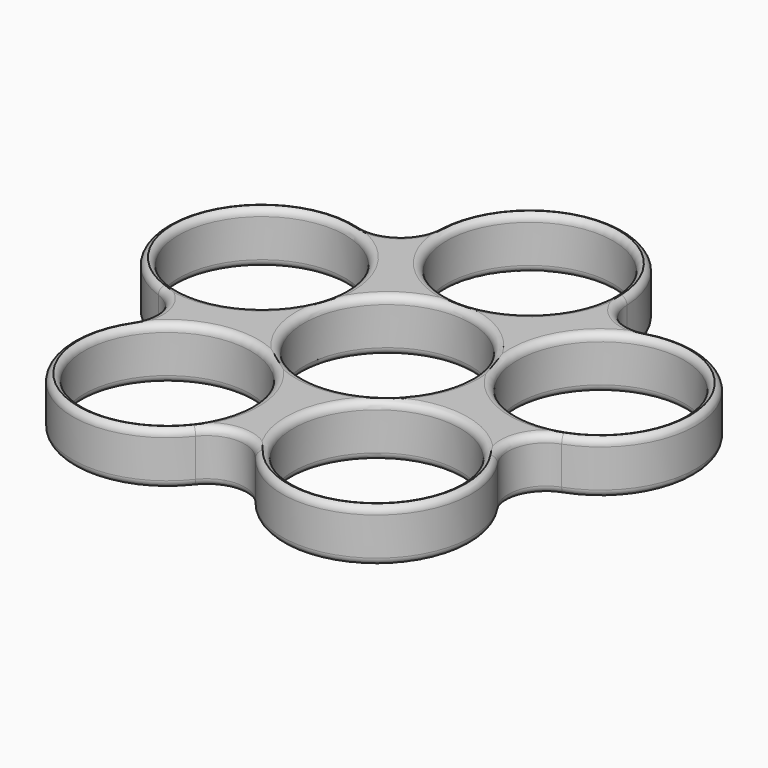
from build123d import *

# Parameters (mm, degrees)
F0_R         = 11
F1_DEPTH     = 7
F2_T3_ANGLE  = 176.2424563909
F2_T6_ANGLE  = 176.2424563909
F2_T45_ANGLE = 104.2424563909
F2_T48_ANGLE = 104.2424563909
F2_T51_ANGLE = 176.2424563909
F2_T54_ANGLE = 104.2424563909
F2_T57_ANGLE = 176.2424563909
F2_T60_ANGLE = 104.2424563909
F2_T63_ANGLE = 176.2424563909
F2_T66_ANGLE = 104.2424563909
F2_T69_ANGLE = 176.2424563909
F2_T72_ANGLE = 104.2424563909
F2_T75_ANGLE = 104.2424563909
F2_T78_ANGLE = 176.2424563909
F2_T81_ANGLE = 104.2424563909
F2_T84_ANGLE = 176.2424563909
F2_T87_ANGLE = 104.2424563909
F2_T90_ANGLE = 176.2424563909
F2_T93_ANGLE = 104.2424563909
F2_T96_ANGLE = 176.2424563909


# Not quite as in the source:
# - a fillet or chamfer that OpenCascade refuses, or shapes differently, is made with other operations: its cross-section is extruded or revolved along the edge and cut away or added


with BuildPart() as f1:
    # F0 (on Top) → F1 (new body)
    with BuildSketch(Plane.XY):
        with BuildLine():
            ThreePointArc((18.8789455733, 19.2703536504), (14.551666288, 20.0286503916), (12.4932803925, 23.9098109739))
            ThreePointArc((12.4932803925, 23.9098109739), (0, 36), (-12.4932803925, 23.9098109739))
            ThreePointArc((-12.4932803925, 23.9098109739), (-14.551666288, 20.0286503916), (-18.8789455733, 19.2703536504))
            ThreePointArc((-18.8789455733, 19.2703536504), (-34.2380345866, 11.1246117975), (-26.6002174869, -4.493277804))
            ThreePointArc((-26.6002174869, -4.493277804), (-23.545090647, -7.6502637008), (-24.1611104286, -12.0000774427))
            ThreePointArc((-24.1611104286, -12.0000774427), (-21.1602690825, -29.1246117975), (-3.9465581225, -26.6868093776))
            ThreePointArc((-3.9465581225, -26.6868093776), (0, -24.7567733816), (3.9465581225, -26.6868093776))
            ThreePointArc((3.9465581225, -26.6868093776), (21.1602690825, -29.1246117975), (24.1611104286, -12.0000774427))
            ThreePointArc((24.1611104286, -12.0000774427), (23.545090647, -7.6502637008), (26.6002174869, -4.493277804))
            ThreePointArc((26.6002174869, -4.493277804), (34.2380345866, 11.1246117975), (18.8789455733, 19.2703536504))
        make_face()
        with Locations((-13.8129534289, -19.0118993678)):
            Circle(F0_R, mode=Mode.SUBTRACT)
        with Locations((13.8129534289, -19.0118993678)):
            Circle(F0_R, mode=Mode.SUBTRACT)
        Circle(F0_R, mode=Mode.SUBTRACT)
        with Locations((-22.3498281329, 7.2618993678)):
            Circle(F0_R, mode=Mode.SUBTRACT)
        with Locations((22.3498281329, 7.2618993678)):
            Circle(F0_R, mode=Mode.SUBTRACT)
        with Locations((0, 23.5)):
            Circle(F0_R, mode=Mode.SUBTRACT)
    extrude(amount=F1_DEPTH)

    # F2: fillet of radius 1 on 14 edges, made by hand


with BuildPart() as f2_tool1:
    # F2_s2 → F2_t3 (revolve)
    with BuildSketch(Plane(origin=(-22.5637579595, 6.5217514376, 0), x_dir=(0, 0, 1), z_dir=(0.9606763426, -0.2776706048, 0))):
        with BuildLine():
            ThreePointArc((6, -13.2704446309), (6.7071067812, -12.9775514121), (7, -12.2704446309))
            Line((7, -12.2704446309), (7, -13.2704446309))
            Line((7, -13.2704446309), (6, -13.2704446309))
        make_face()
    revolve(axis=Axis((-22.3498281329, 7.2618993678, 7), (0, 0, 1)), revolution_arc=F2_T3_ANGLE)


with BuildPart() as f2_tool4:
    # F2_s5 → F2_t6 (revolve)
    with BuildSketch(Plane(origin=(-13.1751388688, -19.4440770122, 0), x_dir=(0, 0, 1), z_dir=(0.560945754, 0.82785256, 0))):
        with BuildLine():
            ThreePointArc((1, -13.2704446309), (0.2928932188, -12.9775514121), (0, -12.2704446309))
            Line((0, -12.2704446309), (0, -13.2704446309))
            Line((0, -13.2704446309), (1, -13.2704446309))
        make_face()
    revolve(axis=Axis((-13.8129534289, -19.0118993678, 0), (0, 0, 1)), revolution_arc=F2_T6_ANGLE)


with BuildPart() as f2_tool7:
    # F2_s8 → F2_t9 (revolve)
    with BuildSketch(Plane.XZ.offset(19.0118993678)):
        with BuildLine():
            ThreePointArc((-2.8129534289, 6), (-2.5200602101, 6.7071067812), (-1.8129534289, 7))
            Line((-1.8129534289, 7), (-2.8129534289, 7))
            Line((-2.8129534289, 7), (-2.8129534289, 6))
        make_face()
    revolve(axis=Axis((-13.8129534289, -19.0118993678, 7), (0, 0, 1)))


with BuildPart() as f2_tool10:
    # F2_s11 → F2_t12 (revolve)
    with BuildSketch(Plane.XZ.offset(-7.2618993678)):
        with BuildLine():
            ThreePointArc((-11.3498281329, 6), (-11.0569349141, 6.7071067812), (-10.3498281329, 7))
            Line((-10.3498281329, 7), (-11.3498281329, 7))
            Line((-11.3498281329, 7), (-11.3498281329, 6))
        make_face()
    revolve(axis=Axis((-22.3498281329, 7.2618993678, 7), (0, 0, 1)))


with BuildPart() as f2_tool13:
    # F2_s14 → F2_t15 (revolve)
    with BuildSketch(Plane.XZ.offset(-23.5)):
        with BuildLine():
            ThreePointArc((11, 1), (11.2928932188, 0.2928932188), (12, 0))
            Line((12, 0), (11, 0))
            Line((11, 0), (11, 1))
        make_face()
    revolve(axis=Axis((0, 23.5, 0), (0, 0, 1)))


with BuildPart() as f2_tool16:
    # F2_s17 → F2_t18 (revolve)
    with BuildSketch(Plane.XZ.offset(-23.5)):
        with BuildLine():
            ThreePointArc((11, 6), (11.2928932188, 6.7071067812), (12, 7))
            Line((12, 7), (11, 7))
            Line((11, 7), (11, 6))
        make_face()
    revolve(axis=Axis((0, 23.5, 7), (0, 0, 1)))


with BuildPart() as f2_tool19:
    # F2_s20 → F2_t21 (revolve)
    with BuildSketch(Plane.XZ.offset(-7.2618993678)):
        with BuildLine():
            ThreePointArc((-11.3498281329, 1), (-11.0569349141, 0.2928932188), (-10.3498281329, 0))
            Line((-10.3498281329, 0), (-11.3498281329, 0))
            Line((-11.3498281329, 0), (-11.3498281329, 1))
        make_face()
    revolve(axis=Axis((-22.3498281329, 7.2618993678, 0), (0, 0, 1)))


with BuildPart() as f2_tool22:
    # F2_s23 → F2_t24 (revolve)
    with BuildSketch(Plane.XZ.offset(19.0118993678)):
        with BuildLine():
            ThreePointArc((-2.8129534289, 1), (-2.5200602101, 0.2928932188), (-1.8129534289, 0))
            Line((-1.8129534289, 0), (-2.8129534289, 0))
            Line((-2.8129534289, 0), (-2.8129534289, 1))
        make_face()
    revolve(axis=Axis((-13.8129534289, -19.0118993678, 0), (0, 0, 1)))


with BuildPart() as f2_tool25:
    # F2_s26 → F2_t27 (revolve)
    with BuildSketch(Plane.XZ):
        with BuildLine():
            ThreePointArc((11, 1), (11.2928932188, 0.2928932188), (12, 0))
            Line((12, 0), (11, 0))
            Line((11, 0), (11, 1))
        make_face()
    revolve(axis=Axis((0, 0, 0), (0, 0, 1)))


with BuildPart() as f2_tool28:
    # F2_s29 → F2_t30 (revolve)
    with BuildSketch(Plane.XZ):
        with BuildLine():
            ThreePointArc((11, 6), (11.2928932188, 6.7071067812), (12, 7))
            Line((12, 7), (11, 7))
            Line((11, 7), (11, 6))
        make_face()
    revolve(axis=Axis((0, 0, 7), (0, 0, 1)))


with BuildPart() as f2_tool31:
    # F2_s32 → F2_t33 (revolve)
    with BuildSketch(Plane.XZ.offset(-7.2618993678)):
        with BuildLine():
            ThreePointArc((33.3498281329, 1), (33.6427213517, 0.2928932188), (34.3498281329, 0))
            Line((34.3498281329, 0), (33.3498281329, 0))
            Line((33.3498281329, 0), (33.3498281329, 1))
        make_face()
    revolve(axis=Axis((22.3498281329, 7.2618993678, 0), (0, 0, 1)))


with BuildPart() as f2_tool34:
    # F2_s35 → F2_t36 (revolve)
    with BuildSketch(Plane.XZ.offset(-7.2618993678)):
        with BuildLine():
            ThreePointArc((33.3498281329, 6), (33.6427213517, 6.7071067812), (34.3498281329, 7))
            Line((34.3498281329, 7), (33.3498281329, 7))
            Line((33.3498281329, 7), (33.3498281329, 6))
        make_face()
    revolve(axis=Axis((22.3498281329, 7.2618993678, 7), (0, 0, 1)))


with BuildPart() as f2_tool37:
    # F2_s38 → F2_t39 (revolve)
    with BuildSketch(Plane.XZ.offset(19.0118993678)):
        with BuildLine():
            ThreePointArc((24.8129534289, 1), (25.1058466477, 0.2928932188), (25.8129534289, 0))
            Line((25.8129534289, 0), (24.8129534289, 0))
            Line((24.8129534289, 0), (24.8129534289, 1))
        make_face()
    revolve(axis=Axis((13.8129534289, -19.0118993678, 0), (0, 0, 1)))


with BuildPart() as f2_tool40:
    # F2_s41 → F2_t42 (revolve)
    with BuildSketch(Plane.XZ.offset(19.0118993678)):
        with BuildLine():
            ThreePointArc((24.8129534289, 6), (25.1058466477, 6.7071067812), (25.8129534289, 7))
            Line((25.8129534289, 7), (24.8129534289, 7))
            Line((24.8129534289, 7), (24.8129534289, 6))
        make_face()
    revolve(axis=Axis((13.8129534289, -19.0118993678, 7), (0, 0, 1)))


with BuildPart() as f2_tool43:
    # F2_s44 → F2_t45 (revolve)
    with BuildSketch(Plane(origin=(-22.0878529604, 7.9864364188, 0), x_dir=(0, 0, 1), z_dir=(-0.9404141737, 0.3400311483, 0))):
        with BuildLine():
            ThreePointArc((1, -13.2704446309), (0.2928932188, -12.9775514121), (0, -12.2704446309))
            Line((0, -12.2704446309), (0, -13.2704446309))
            Line((0, -13.2704446309), (1, -13.2704446309))
        make_face()
    revolve(axis=Axis((-28.3003732285, -9.1953486727, 0), (0, 0, -1)), revolution_arc=F2_T45_ANGLE)


with BuildPart() as f2_tool46:
    # F2_s47 → F2_t48 (revolve)
    with BuildSketch(Plane(origin=(-14.4210743321, -18.538851911, 0), x_dir=(0, 0, 1), z_dir=(-0.6139928008, -0.7893116245, 0))):
        with BuildLine():
            ThreePointArc((1, -13.2704446309), (0.2928932188, -12.9775514121), (0, -12.2704446309))
            Line((0, -12.2704446309), (0, -13.2704446309))
            Line((0, -13.2704446309), (1, -13.2704446309))
        make_face()
    revolve(axis=Axis((0, -29.7567733816, 0), (0, 0, -1)), revolution_arc=F2_T48_ANGLE)


with BuildPart() as f2_tool49:
    # F2_s50 → F2_t51 (revolve)
    with BuildSketch(Plane(origin=(14.4210743321, -18.538851911, 0), x_dir=(0, 0, 1), z_dir=(-0.6139928008, 0.7893116245, 0))):
        with BuildLine():
            ThreePointArc((1, -13.2704446309), (0.2928932188, -12.9775514121), (0, -12.2704446309))
            Line((0, -12.2704446309), (0, -13.2704446309))
            Line((0, -13.2704446309), (1, -13.2704446309))
        make_face()
    revolve(axis=Axis((13.8129534289, -19.0118993678, 0), (0, 0, 1)), revolution_arc=F2_T51_ANGLE)


with BuildPart() as f2_tool52:
    # F2_s53 → F2_t54 (revolve)
    with BuildSketch(Plane(origin=(13.1751388688, -19.4440770122, 0), x_dir=(0, 0, 1), z_dir=(0.560945754, -0.82785256, 0))):
        with BuildLine():
            ThreePointArc((1, -13.2704446309), (0.2928932188, -12.9775514121), (0, -12.2704446309))
            Line((0, -12.2704446309), (0, -13.2704446309))
            Line((0, -13.2704446309), (1, -13.2704446309))
        make_face()
    revolve(axis=Axis((28.3003732285, -9.1953486727, 0), (0, 0, -1)), revolution_arc=F2_T54_ANGLE)


with BuildPart() as f2_tool55:
    # F2_s56 → F2_t57 (revolve)
    with BuildSketch(Plane(origin=(22.0878529604, 7.9864364188, 0), x_dir=(0, 0, 1), z_dir=(-0.9404141737, -0.3400311483, 0))):
        with BuildLine():
            ThreePointArc((1, -13.2704446309), (0.2928932188, -12.9775514121), (0, -12.2704446309))
            Line((0, -12.2704446309), (0, -13.2704446309))
            Line((0, -13.2704446309), (1, -13.2704446309))
        make_face()
    revolve(axis=Axis((22.3498281329, 7.2618993678, 0), (0, 0, 1)), revolution_arc=F2_T57_ANGLE)


with BuildPart() as f2_tool58:
    # F2_s59 → F2_t60 (revolve)
    with BuildSketch(Plane(origin=(22.5637579595, 6.5217514376, 0), x_dir=(0, 0, 1), z_dir=(0.9606763426, 0.2776706048, 0))):
        with BuildLine():
            ThreePointArc((1, -13.2704446309), (0.2928932188, -12.9775514121), (0, -12.2704446309))
            Line((0, -12.2704446309), (0, -13.2704446309))
            Line((0, -13.2704446309), (1, -13.2704446309))
        make_face()
    revolve(axis=Axis((17.4905925495, 24.0737353635, 0), (0, 0, -1)), revolution_arc=F2_T60_ANGLE)


with BuildPart() as f2_tool61:
    # F2_s62 → F2_t63 (revolve)
    with BuildSketch(Plane(origin=(-0.7700304641, 23.4747410668, 0), x_dir=(0, 0, 1), z_dir=(0.0327848779, -0.9994624314, 0))):
        with BuildLine():
            ThreePointArc((1, -13.2704446309), (0.2928932188, -12.9775514121), (0, -12.2704446309))
            Line((0, -12.2704446309), (0, -13.2704446309))
            Line((0, -13.2704446309), (1, -13.2704446309))
        make_face()
    revolve(axis=Axis((0, 23.5, 0), (0, 0, 1)), revolution_arc=F2_T63_ANGLE)


with BuildPart() as f2_tool64:
    # F2_s65 → F2_t66 (revolve)
    with BuildSketch(Plane(origin=(0.7700304641, 23.4747410668, 0), x_dir=(0, 0, 1), z_dir=(0.0327848779, 0.9994624314, 0))):
        with BuildLine():
            ThreePointArc((1, -13.2704446309), (0.2928932188, -12.9775514121), (0, -12.2704446309))
            Line((0, -12.2704446309), (0, -13.2704446309))
            Line((0, -13.2704446309), (1, -13.2704446309))
        make_face()
    revolve(axis=Axis((-17.4905925495, 24.0737353635, 0), (0, 0, -1)), revolution_arc=F2_T66_ANGLE)


with BuildPart() as f2_tool67:
    # F2_s68 → F2_t69 (revolve)
    with BuildSketch(Plane(origin=(-22.5637579595, 6.5217514376, 0), x_dir=(0, 0, 1), z_dir=(0.9606763426, -0.2776706048, 0))):
        with BuildLine():
            ThreePointArc((1, -13.2704446309), (0.2928932188, -12.9775514121), (0, -12.2704446309))
            Line((0, -12.2704446309), (0, -13.2704446309))
            Line((0, -13.2704446309), (1, -13.2704446309))
        make_face()
    revolve(axis=Axis((-22.3498281329, 7.2618993678, 0), (0, 0, 1)), revolution_arc=F2_T69_ANGLE)


with BuildPart() as f2_tool70:
    # F2_s71 → F2_t72 (revolve)
    with BuildSketch(Plane(origin=(0.7700304641, 23.4747410668, 0), x_dir=(0, 0, 1), z_dir=(0.0327848779, 0.9994624314, 0))):
        with BuildLine():
            ThreePointArc((6, -13.2704446309), (6.7071067812, -12.9775514121), (7, -12.2704446309))
            Line((7, -12.2704446309), (7, -13.2704446309))
            Line((7, -13.2704446309), (6, -13.2704446309))
        make_face()
    revolve(axis=Axis((-17.4905925495, 24.0737353635, 7), (0, 0, -1)), revolution_arc=F2_T72_ANGLE)


with BuildPart() as f2_tool73:
    # F2_s74 → F2_t75 (revolve)
    with BuildSketch(Plane(origin=(-22.0878529604, 7.9864364188, 0), x_dir=(0, 0, 1), z_dir=(-0.9404141737, 0.3400311483, 0))):
        with BuildLine():
            ThreePointArc((6, -13.2704446309), (6.7071067812, -12.9775514121), (7, -12.2704446309))
            Line((7, -12.2704446309), (7, -13.2704446309))
            Line((7, -13.2704446309), (6, -13.2704446309))
        make_face()
    revolve(axis=Axis((-28.3003732285, -9.1953486727, 7), (0, 0, -1)), revolution_arc=F2_T75_ANGLE)


with BuildPart() as f2_tool76:
    # F2_s77 → F2_t78 (revolve)
    with BuildSketch(Plane(origin=(-13.1751388688, -19.4440770122, 0), x_dir=(0, 0, 1), z_dir=(0.560945754, 0.82785256, 0))):
        with BuildLine():
            ThreePointArc((6, -13.2704446309), (6.7071067812, -12.9775514121), (7, -12.2704446309))
            Line((7, -12.2704446309), (7, -13.2704446309))
            Line((7, -13.2704446309), (6, -13.2704446309))
        make_face()
    revolve(axis=Axis((-13.8129534289, -19.0118993678, 7), (0, 0, 1)), revolution_arc=F2_T78_ANGLE)


with BuildPart() as f2_tool79:
    # F2_s80 → F2_t81 (revolve)
    with BuildSketch(Plane(origin=(-14.4210743321, -18.538851911, 0), x_dir=(0, 0, 1), z_dir=(-0.6139928008, -0.7893116245, 0))):
        with BuildLine():
            ThreePointArc((6, -13.2704446309), (6.7071067812, -12.9775514121), (7, -12.2704446309))
            Line((7, -12.2704446309), (7, -13.2704446309))
            Line((7, -13.2704446309), (6, -13.2704446309))
        make_face()
    revolve(axis=Axis((0, -29.7567733816, 7), (0, 0, -1)), revolution_arc=F2_T81_ANGLE)


with BuildPart() as f2_tool82:
    # F2_s83 → F2_t84 (revolve)
    with BuildSketch(Plane(origin=(14.4210743321, -18.538851911, 0), x_dir=(0, 0, 1), z_dir=(-0.6139928008, 0.7893116245, 0))):
        with BuildLine():
            ThreePointArc((6, -13.2704446309), (6.7071067812, -12.9775514121), (7, -12.2704446309))
            Line((7, -12.2704446309), (7, -13.2704446309))
            Line((7, -13.2704446309), (6, -13.2704446309))
        make_face()
    revolve(axis=Axis((13.8129534289, -19.0118993678, 7), (0, 0, 1)), revolution_arc=F2_T84_ANGLE)


with BuildPart() as f2_tool85:
    # F2_s86 → F2_t87 (revolve)
    with BuildSketch(Plane(origin=(13.1751388688, -19.4440770122, 0), x_dir=(0, 0, 1), z_dir=(0.560945754, -0.82785256, 0))):
        with BuildLine():
            ThreePointArc((6, -13.2704446309), (6.7071067812, -12.9775514121), (7, -12.2704446309))
            Line((7, -12.2704446309), (7, -13.2704446309))
            Line((7, -13.2704446309), (6, -13.2704446309))
        make_face()
    revolve(axis=Axis((28.3003732285, -9.1953486727, 7), (0, 0, -1)), revolution_arc=F2_T87_ANGLE)


with BuildPart() as f2_tool88:
    # F2_s89 → F2_t90 (revolve)
    with BuildSketch(Plane(origin=(22.0878529604, 7.9864364188, 0), x_dir=(0, 0, 1), z_dir=(-0.9404141737, -0.3400311483, 0))):
        with BuildLine():
            ThreePointArc((6, -13.2704446309), (6.7071067812, -12.9775514121), (7, -12.2704446309))
            Line((7, -12.2704446309), (7, -13.2704446309))
            Line((7, -13.2704446309), (6, -13.2704446309))
        make_face()
    revolve(axis=Axis((22.3498281329, 7.2618993678, 7), (0, 0, 1)), revolution_arc=F2_T90_ANGLE)


with BuildPart() as f2_tool91:
    # F2_s92 → F2_t93 (revolve)
    with BuildSketch(Plane(origin=(22.5637579595, 6.5217514376, 0), x_dir=(0, 0, 1), z_dir=(0.9606763426, 0.2776706048, 0))):
        with BuildLine():
            ThreePointArc((6, -13.2704446309), (6.7071067812, -12.9775514121), (7, -12.2704446309))
            Line((7, -12.2704446309), (7, -13.2704446309))
            Line((7, -13.2704446309), (6, -13.2704446309))
        make_face()
    revolve(axis=Axis((17.4905925495, 24.0737353635, 7), (0, 0, -1)), revolution_arc=F2_T93_ANGLE)


with BuildPart() as f2_tool94:
    # F2_s95 → F2_t96 (revolve)
    with BuildSketch(Plane(origin=(-0.7700304641, 23.4747410668, 0), x_dir=(0, 0, 1), z_dir=(0.0327848779, -0.9994624314, 0))):
        with BuildLine():
            ThreePointArc((6, -13.2704446309), (6.7071067812, -12.9775514121), (7, -12.2704446309))
            Line((7, -12.2704446309), (7, -13.2704446309))
            Line((7, -13.2704446309), (6, -13.2704446309))
        make_face()
    revolve(axis=Axis((0, 23.5, 7), (0, 0, 1)), revolution_arc=F2_T96_ANGLE)


with BuildPart() as f1_1:
    add(f1.part)

    # F2_t97: cut F2_tool1, F2_tool4, F2_tool7, F2_tool10, F2_tool13, F2_tool16, F2_tool19, F2_tool22, F2_tool25, F2_tool28, F2_tool31, F2_tool34, F2_tool37, F2_tool40, F2_tool43, F2_tool46, F2_tool49, F2_tool52, F2_tool55, F2_tool58, F2_tool61, F2_tool64, F2_tool67, F2_tool70, F2_tool73, F2_tool76, F2_tool79, F2_tool82, F2_tool85, F2_tool88, F2_tool91, F2_tool94
    add([f2_tool1.part, f2_tool4.part, f2_tool7.part, f2_tool10.part, f2_tool13.part, f2_tool16.part, f2_tool19.part, f2_tool22.part, f2_tool25.part, f2_tool28.part, f2_tool31.part, f2_tool34.part, f2_tool37.part, f2_tool40.part, f2_tool43.part, f2_tool46.part, f2_tool49.part, f2_tool52.part, f2_tool55.part, f2_tool58.part, f2_tool61.part, f2_tool64.part, f2_tool67.part, f2_tool70.part, f2_tool73.part, f2_tool76.part, f2_tool79.part, f2_tool82.part, f2_tool85.part, f2_tool88.part, f2_tool91.part, f2_tool94.part], mode=Mode.SUBTRACT)


solid = f1_1.part
